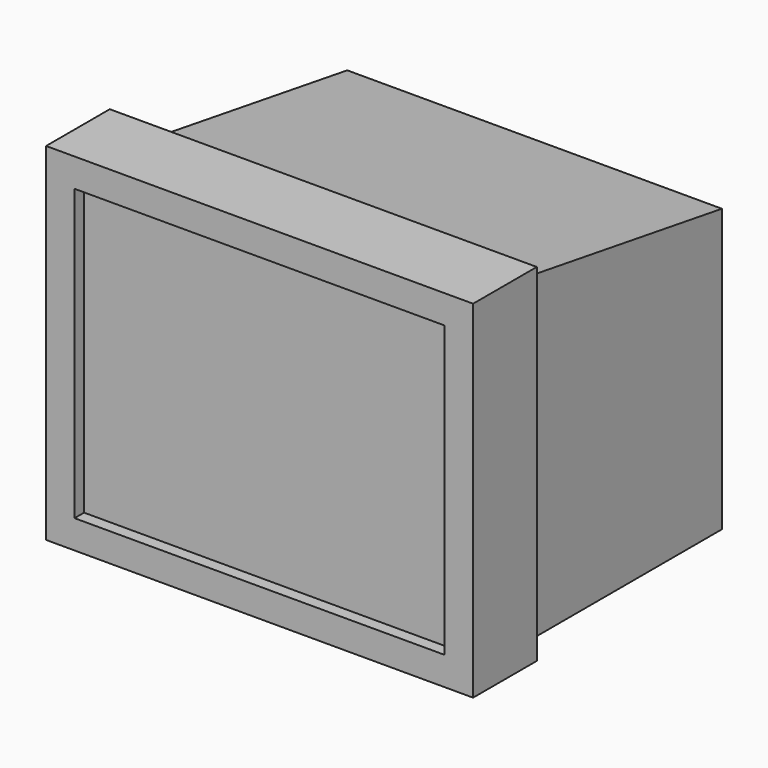
from build123d import *

# Parameters (mm, degrees)
F0_W         = 95.3711643815
F0_H         = 77.4655118585
F1_DEPTH     = 10.16
F2_T         = -6.35
F3_DEPTH     = 5.588
F4_DEPTH     = 3.8735
F5_DEPTH     = 0.5715
F6_DEPTH     = 7.62
F7_W         = 83.6853682995
F7_H         = 57.4865713716
F7_H_2       = 9.9894702435
F8_DEPTH     = 58.9915
F9_DEPTH     = 5.715
F10_T4_DEPTH = 413.7319634586


# Not quite as in the source:
# - a fillet or chamfer that OpenCascade refuses, or shapes differently, is made with other operations: its cross-section is extruded or revolved along the edge and cut away or added


with BuildPart() as f1:
    # F0 (on Front) → F1 (new body)
    with BuildSketch(Plane.XZ):
        Rectangle(F0_W, F0_H)
    extrude(amount=-F1_DEPTH)

    # F2
    f2_openings = [f1.faces().sort_by_distance(p)[0] for p in [
        (0, 0, 0),
    ]]
    offset(amount=F2_T, openings=f2_openings)

    # F3 (add): a face of the model
    f3_faces = [f1.faces().sort_by_distance(p)[0] for p in [
        (0, 3.81, 0),
    ]]
    extrude(f3_faces, amount=F3_DEPTH)

    # F4 (cut): a face of the model
    f4_faces = [f1.faces().sort_by_distance(p)[0] for p in [
        (0, -1.778, 0),
    ]]
    extrude(f4_faces, amount=-F4_DEPTH, mode=Mode.SUBTRACT)

    # F5 (cut): a face of the model
    f5_faces = [f1.faces().sort_by_distance(p)[0] for p in [
        (0, 2.0955, 0),
    ]]
    extrude(f5_faces, amount=-F5_DEPTH, mode=Mode.SUBTRACT)

    # F6 (add): a face of the model
    f6_faces = [f1.faces().sort_by_distance(p)[0] for p in [
        (0, 10.16, 0),
    ]]
    extrude(f6_faces, amount=F6_DEPTH)

    # F7 (on face) → F8 (join)
    with BuildSketch(Plane(origin=(0, 17.78, 0), x_dir=(-1, 0, 0), z_dir=(0, 1, 0))):
        Rectangle(F7_W, F7_H)
        with Locations((0, -33.7380208075)):
            Rectangle(F7_W, F7_H_2)
    extrude(amount=F8_DEPTH)

    # F9 (add): a face of the model
    f9_faces = [f1.faces().sort_by_distance(p)[0] for p in [
        (0, 47.27575, 28.7432856858),
    ]]
    extrude(f9_faces, amount=F9_DEPTH)

    # F10: chamfer of 63.5 x 10.16 on 1 edges, made by hand


with BuildPart() as f10_tool2:
    # F10_s3 → F10_t4 (new body)
    with BuildSketch(Plane.YZ.offset(-206.8659817293)):
        Polygon((13.2715, 34.4582856858), (76.7715, 24.2982856858), (76.7715, 34.4582856858), align=None)
    extrude(amount=F10_T4_DEPTH)

    split(bisect_by=Plane.XZ.offset(-17.78), keep=Keep.BOTTOM)


with BuildPart() as f1_1:
    add(f1.part)

    # F10_t1: cut F10_tool2
    add(f10_tool2.part, mode=Mode.SUBTRACT)


solid = f1_1.part
